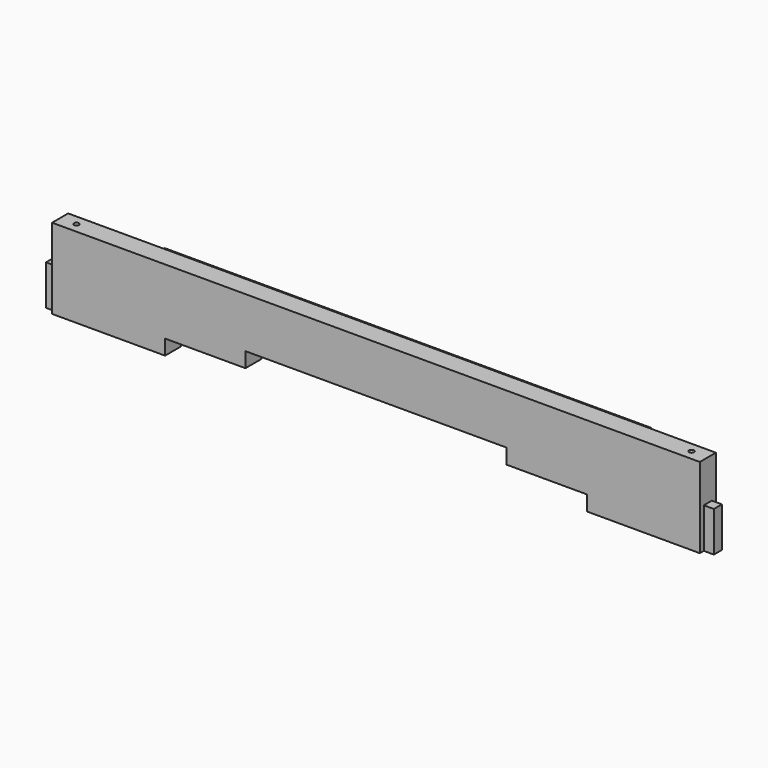
from build123d import *

# Parameters (mm, degrees)
F0_W      = 819.15
F0_H      = 101.6
F1_DEPTH  = 25.4
F2_R      = 4.5640625
F3_DEPTH  = 50.8
F4_R      = 12.7
F5_DEPTH  = 19.05
F7_DEPTH  = 25.4
F9_D      = 6.35
F9_DEPTH  = 12.7
F9_TIP    = 1.9077324654
F10_W     = 12.7
F10_H     = 12.7
F11_DEPTH = 50.8
F12_W     = 615.95
F12_H     = 25.4
F13_DEPTH = 25.4


# Not quite as in the source:
# - a feature names something its author has since deleted; it is built from what else it names


with BuildPart() as f1:
    # F0 (on Front) → F1 (new body)
    with BuildSketch(Plane.XZ):
        with Locations((409.575, 50.8)):
            Rectangle(F0_W, F0_H)
    extrude(amount=F1_DEPTH)

    # F2 (on face) → F3 (cut)
    with BuildSketch(Plane(origin=(0, 0, 0), x_dir=(0, -1, 0), z_dir=(-1, 0, 0))):
        with Locations((12.7, 76.2)):
            Circle(F2_R)
    extrude(amount=-F3_DEPTH, mode=Mode.SUBTRACT)

    # F4 (on Front) → F5 (cut)
    with BuildSketch(Plane.XZ):
        with Locations((765.175, 76.2)):
            Circle(F4_R)
        with Locations((53.975, 76.2)):
            Circle(F4_R)
    extrude(amount=F5_DEPTH, mode=Mode.SUBTRACT)

    # F6 (on face) → F7 (cut, through all)
    with BuildSketch(Plane(origin=(0, 0, 0), x_dir=(-1, 0, 0), z_dir=(0, 1, 0))):
        Polygon((-676.275, 19.05), (-676.275, 0), (-142.875, 0), (-142.875, 19.05), (-244.475, 19.05), (-244.475, 38.1), (-574.675, 38.1), (-574.675, 19.05), align=None)
    extrude(amount=-F7_DEPTH, mode=Mode.SUBTRACT)

    # F9
    with Locations(Plane.XY.offset(101.6)):
        with Locations((20.6375, -12.7), (798.5125, -12.7)):
            Hole(F9_D / 2, depth=F9_DEPTH)
            with Locations((0, 0, -(F9_DEPTH + F9_TIP / 2))):  # 118° drill point
                Cone(0, F9_D / 2, F9_TIP, mode=Mode.SUBTRACT)

    # F10 (on Top) → F11 (join)
    with BuildSketch(Plane.XY):
        with Locations((-6.35, -12.7)):
            Rectangle(F10_W, F10_H)
        with Locations((825.5, -12.7)):
            Rectangle(F10_W, F10_H)
    extrude(amount=F11_DEPTH)

    # F12 (on face) → F13 (join)
    with BuildSketch(Plane(origin=(0, 0, 0), x_dir=(-1, 0, 0), z_dir=(0, 1, 0))):
        with Locations((-409.575, 73.025)):
            Rectangle(F12_W, F12_H)
    extrude(amount=F13_DEPTH)


solid = f1.part
